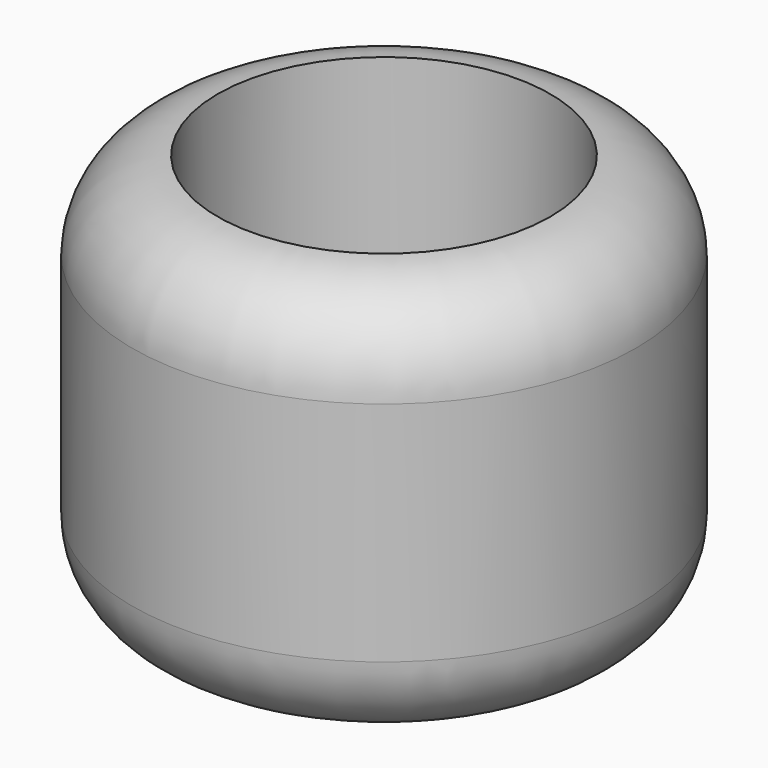
from build123d import *

# Parameters (mm, degrees)
F0_R     = 14.400864616
F0_R_2   = 9.5
F1_DEPTH = 23


# Not quite as in the source:
# - a fillet or chamfer that OpenCascade refuses, or shapes differently, is made with other operations: its cross-section is extruded or revolved along the edge and cut away or added


with BuildPart() as f1:
    # F0 (on Top) → F1 (new body)
    with BuildSketch(Plane.XY):
        Circle(F0_R)
        Circle(F0_R_2, mode=Mode.SUBTRACT)
    extrude(amount=F1_DEPTH)

    # F2: fillet of radius 5.08 on 3 edges, made by hand

    # F2_s1 → F2_t2 (revolve, cut)
    with BuildSketch(Plane.XZ):
        with BuildLine():
            ThreePointArc((14.401264616, 5.0777727304), (12.976092899, 1.5489594887), (9.5000141785, -0.0003997486))
            Line((9.5000141785, -0.0003997486), (9.5180257033, -0.5082169965))
            ThreePointArc((9.5180257033, -0.5082169965), (11.9504393973, -0.5081365685), (14.400864616, -0.5081365685))
            Line((14.400864616, -0.5081365685), (14.9090011846, 0))
            ThreePointArc((14.9090011846, 0), (14.9090011846, 2.5388863652), (14.9094011846, 5.0777727304))
            Line((14.9094011846, 5.0777727304), (14.401264616, 5.0777727304))
        make_face()
    revolve(axis=Axis((0, 0, 0), (0, 0, 1)), mode=Mode.SUBTRACT)

    # F2_s3 → F2_t4 (revolve, cut)
    with BuildSketch(Plane.XZ):
        with BuildLine():
            ThreePointArc((14.401264616, 17.9222272696), (12.976092899, 21.4510405113), (9.5000141785, 23.0003997486))
            Line((9.5000141785, 23.0003997486), (9.5180257033, 23.5082169965))
            ThreePointArc((9.5180257033, 23.5082169965), (11.9504393973, 23.5081365685), (14.400864616, 23.5081365685))
            Line((14.400864616, 23.5081365685), (14.9090011846, 23))
            ThreePointArc((14.9090011846, 23), (14.9090011846, 20.4611136348), (14.9094011846, 17.9222272696))
            Line((14.9094011846, 17.9222272696), (14.401264616, 17.9222272696))
        make_face()
    revolve(axis=Axis((0, 0, 23), (0, 0, 1)), mode=Mode.SUBTRACT)


solid = f1.part
